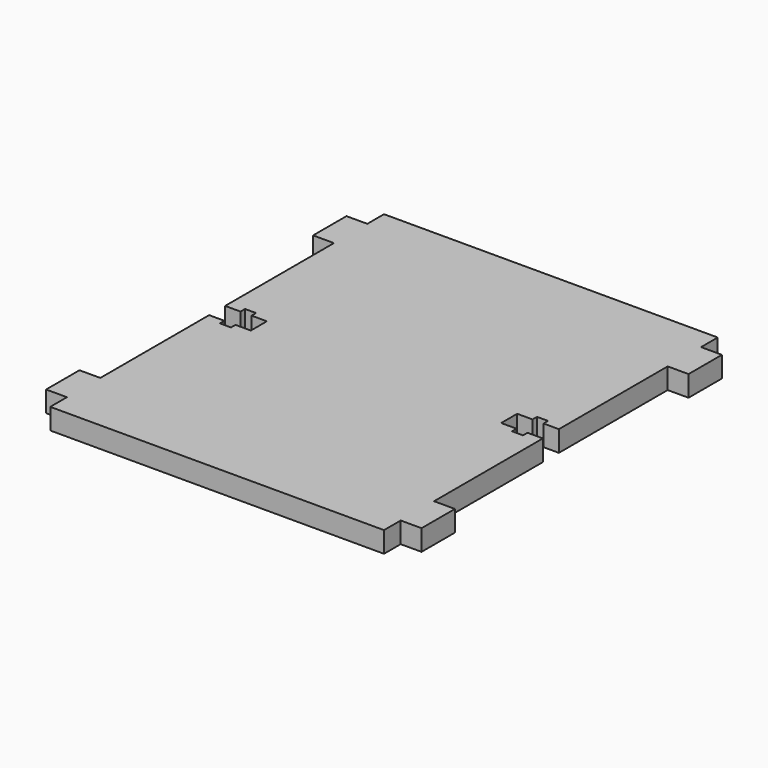
from build123d import *

# Parameters (mm, degrees)
F1_DEPTH = 3.175


# Not quite as in the source:
# - a length typed as a fraction of an inch, garbled in the dataset ("3 / 203.2 mm" for 3/8 in), is restored


with BuildPart() as f1:
    # F0 (on Top) → F1 (new body)
    with BuildSketch(Plane.XY):
        Polygon((25.4, 28.575), (25.4, 31.75), (-25.4, 31.75), (-25.4, 28.575), (-28.575, 28.575), (-28.575, 22.225), (-25.4, 22.225), (-25.4, 1.524), (-23.0632, 1.524), (-23.0632, 2.38125), (-21.3868, 2.38125), (-21.3868, 1.524), (-19.05, 1.524), (-19.05, -1.524), (-21.3868, -1.524), (-21.3868, -2.38125), (-23.0632, -2.38125), (-23.0632, -1.524), (-25.4, -1.524), (-25.4, -22.225), (-28.575, -22.225), (-28.575, -28.575), (-25.4, -28.575), (-25.4, -31.75), (25.4, -31.75), (25.4, -28.575), (28.575, -28.575), (28.575, -22.225), (25.4, -22.225), (25.4, -1.524), (23.0632, -1.524), (23.0632, -2.38125), (21.3868, -2.38125), (21.3868, -1.524), (19.05, -1.524), (19.05, 1.524), (21.3868, 1.524), (21.3868, 2.38125), (23.0632, 2.38125), (23.0632, 1.524), (25.4, 1.524), (25.4, 22.225), (28.575, 22.225), (28.575, 28.575), align=None)
    extrude(amount=F1_DEPTH)


solid = f1.part
